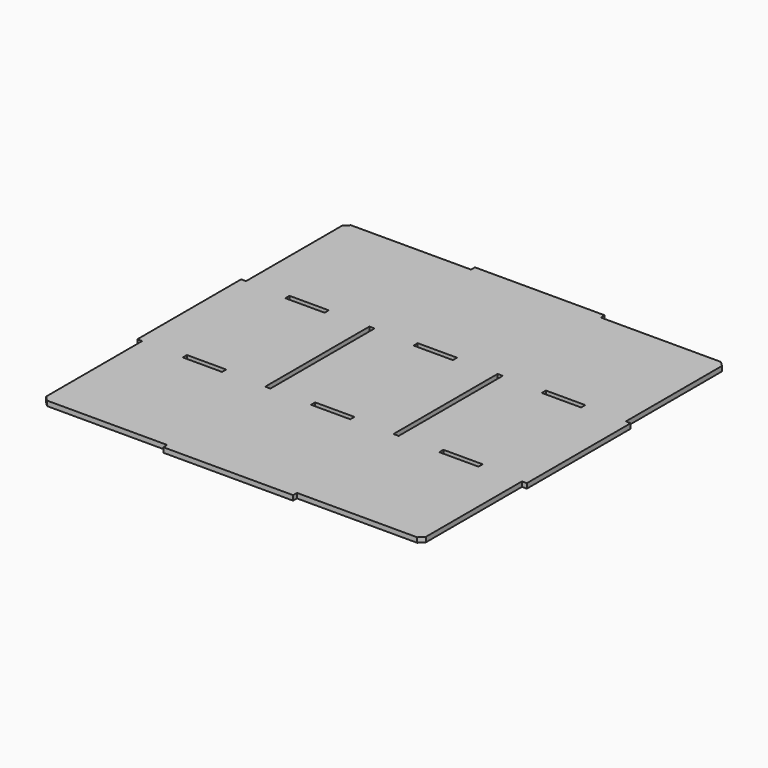
from build123d import *

# Parameters (mm, degrees)
F1_DEPTH = 3
F2_SIZE  = 3
F3_W     = 3.2
F3_H     = 80.2
F4_DEPTH = 3.001
F5_W     = 24.2
F5_H     = 3.2
F6_DEPTH = 3.001
F7_W     = 24.2
F7_H     = 3.2
F8_DEPTH = 3.001


# Not quite as in the source:
# - a pattern or mirror of a feature is missing from the dataset's text; its kind, count and spacing are read off the source's solid


with BuildPart() as f1:
    # F0 (on Top) → F1 (new body)
    with BuildSketch(Plane.XY):
        Polygon((117, 40), (117, 117), (40, 117), (40, 120), (-40, 120), (-40, 117), (-117, 117), (-117, 40), (-120, 40), (-120, -40), (-117, -40), (-117, -117), (-40, -117), (-40, -120), (40, -120), (40, -117), (117, -117), (117, -40), (120, -40), (120, 40), align=None)
    extrude(amount=F1_DEPTH)

    # F2
    f2_edges = [f1.edges().sort_by_distance(p)[0] for p in [
        (117, -117, 1.5),
        (-117, 117, 1.5),
        (117, 117, 1.5),
        (-117, -117, 1.5),
    ]]
    chamfer(f2_edges, length=F2_SIZE)

    # F3 (on face) → F4 (cut, through all)
    with BuildSketch(Plane.XY.offset(3)):
        with Locations((-39.5, 0)):
            Rectangle(F3_W, F3_H)
    f4 = extrude(amount=-F4_DEPTH, mode=Mode.SUBTRACT)

    # F4_copies: F4 across plane
    add(f4.mirror(Plane(origin=(0, 0, 0), x_dir=(0, 0, 1), z_dir=(1, 0, 0))), mode=Mode.SUBTRACT)

    # F5 (on face) → F6 (cut, through all)
    with BuildSketch(Plane.XY.offset(3)):
        with Locations((-79, 39.5)):
            Rectangle(F5_W, F5_H)
        with Locations((-79, -39.5)):
            Rectangle(F5_W, F5_H)
    f6 = extrude(amount=-F6_DEPTH, mode=Mode.SUBTRACT)

    # F6_copies: F6 across plane
    add(f6.mirror(Plane(origin=(0, 0, 0), x_dir=(0, 0, 1), z_dir=(1, 0, 0))), mode=Mode.SUBTRACT)

    # F7 (on face) → F8 (cut, through all)
    with BuildSketch(Plane.XY.offset(3)):
        with Locations((0, 39.5)):
            Rectangle(F7_W, F7_H)
        with Locations((0, -39.5)):
            Rectangle(F7_W, F7_H)
    extrude(amount=-F8_DEPTH, mode=Mode.SUBTRACT)


solid = f1.part
